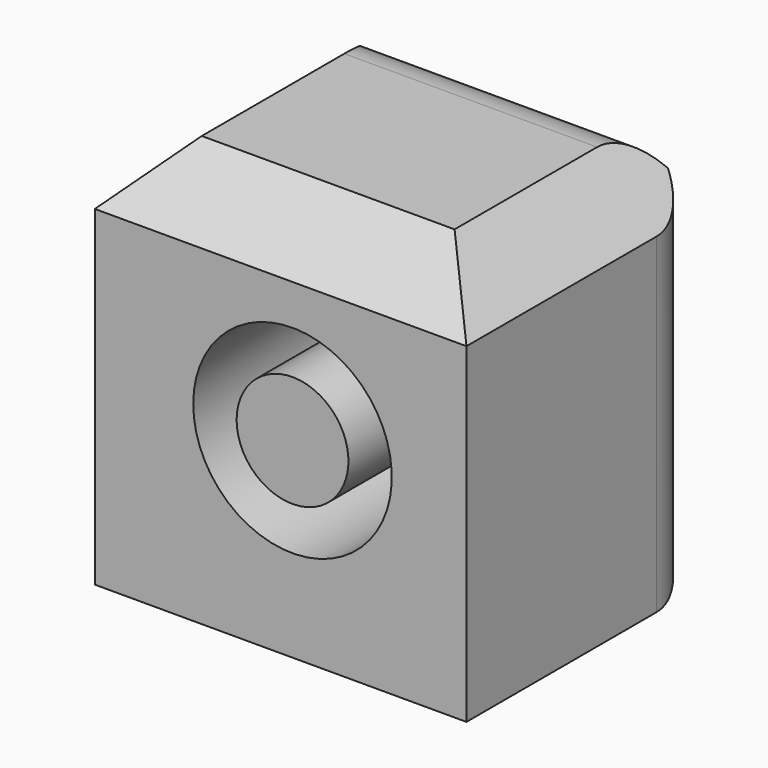
from build123d import *

# Parameters (mm, degrees)
F0_W        = 31.7861549556
F0_H        = 33.3705097437
F1_DEPTH    = 25.4
F2_R        = 8.4913873206
F2_R_2      = 4.7802100494
F3_DEPTH    = 25.401
F4_R        = 5.08
F5_T1_DEPTH = 57.9144541134
F5_T3_DEPTH = 46.4482991577


# Not quite as in the source:
# - a fillet or chamfer that OpenCascade refuses, or shapes differently, is made with other operations: its cross-section is extruded or revolved along the edge and cut away or added


with BuildPart() as f1:
    # F0 (on Front) → F1 (new body)
    with BuildSketch(Plane.XZ):
        with Locations((15.8930774778, 16.6852548718)):
            Rectangle(F0_W, F0_H)
    extrude(amount=F1_DEPTH)

    # F2 (on face) → F3 (cut, through all)
    with BuildSketch(Plane(origin=(0, 0, 0), x_dir=(-1, 0, 0), z_dir=(0, 1, 0))):
        with Locations((-16.9071946293, 16.3528900594)):
            Circle(F2_R)
        with Locations((-16.9071946293, 16.3528900594)):
            Circle(F2_R_2, mode=Mode.SUBTRACT)
    extrude(amount=-F3_DEPTH, mode=Mode.SUBTRACT)

    # F4
    f4_edges = [f1.edges().sort_by_distance(p)[0] for p in [
        (15.893077, 0, 33.37051),
        (0, 0, 16.685255),
        (15.893077, 0, 0),
        (31.786155, 0, 16.685255),
    ]]
    fillet(f4_edges, radius=F4_R)

    # F5: chamfer of 5.08 on 4 edges, made by hand

    # F5_s2 → F5_t1 (cut)
    with BuildSketch(Plane.YZ.offset(-13.0641495789)):
        Polygon((-20.32, 33.3705097437), (-25.4, 28.2905097437), (-25.4, 33.3705097437), align=None)
    extrude(amount=F5_T1_DEPTH, mode=Mode.SUBTRACT)

    # F5_s4 → F5_t3 (cut)
    with BuildSketch(Plane.XZ.offset(-7.9841495789)):
        Polygon((26.7061549556, 33.3705097437), (31.7861549556, 28.2905097437), (31.7861549556, 33.3705097437), align=None)
        Polygon((0, 28.2905097437), (5.08, 33.3705097437), (0, 33.3705097437), align=None)
    extrude(amount=F5_T3_DEPTH, mode=Mode.SUBTRACT)


solid = f1.part
